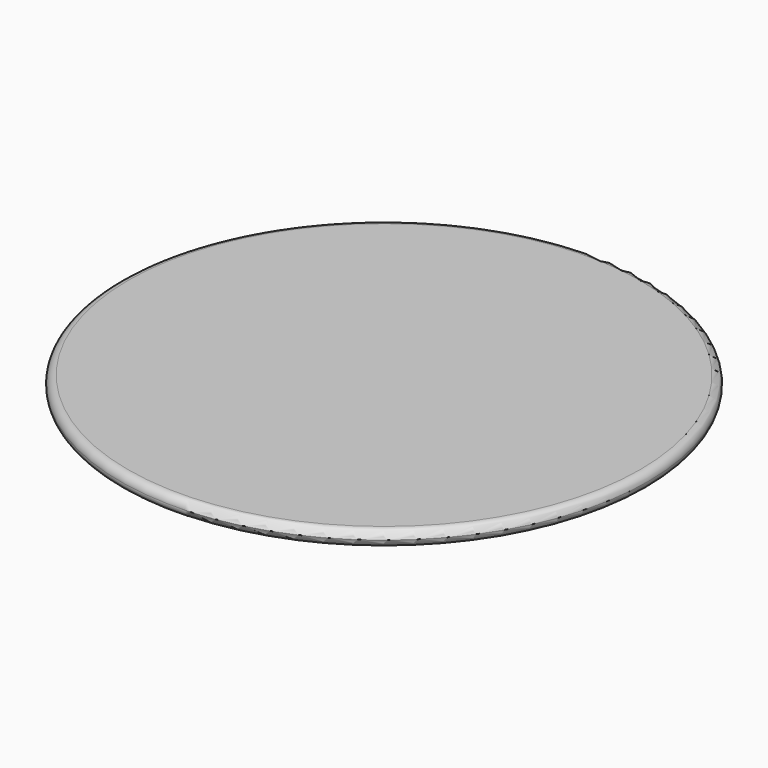
from build123d import *

# Parameters (mm, degrees)
F0_R     = 33.5
F1_DEPTH = 2
F2_R     = 0.99999


# Not quite as in the source:
# - a fillet or chamfer is up to 0.001 mm smaller than in the source, because OpenCascade refuses the exact size


with BuildPart() as f1:
    # F0 (on Top) → F1 (new body)
    with BuildSketch(Plane.XY):
        Circle(F0_R)
    extrude(amount=F1_DEPTH)

    # F2 (radius 1 in the source; OpenCascade refuses exactly that, so slightly less here)
    f2_edges = [f1.edges().sort_by_distance(p)[0] for p in [
        (-33.5, 0, 2),
        (-33.5, 0, 0),
    ]]
    fillet(f2_edges, radius=F2_R)


solid = f1.part
